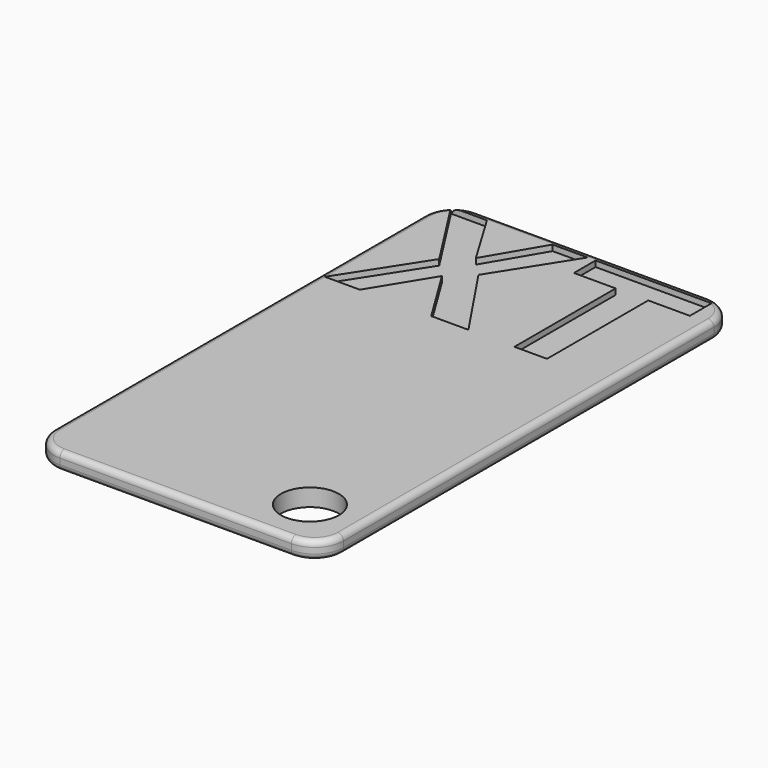
from build123d import *

# Parameters (mm, degrees)
F0_W         = 90
F0_H         = 50
F1_DEPTH     = 3
F2_R         = 1
F3_T1_DEPTH  = 3
F3_T4_ANGLE  = 90
F3_T6_ANGLE  = 90
F3_T8_ANGLE  = 90
F3_T10_ANGLE = 90
F3_T12_ANGLE = 90
F3_T14_ANGLE = 90
F3_T16_ANGLE = 90
F3_T18_ANGLE = 90
F5_ANGLE     = 90
F6_TEXT_SIZE = 37.1822803195
F7_DEPTH     = 1
F8_R         = 5
F9_DEPTH     = 3


# Not quite as in the source:
# - a fillet or chamfer that OpenCascade refuses, or shapes differently, is made with other operations: its cross-section is extruded or revolved along the edge and cut away or added
# - Text() gives the source's letters only with a copy of the font that has no kerning and outlines rounded to 1/6400 em; it was checked with that copy


with BuildPart() as f1:
    # F0 (on Top) → F1 (new body)
    with BuildSketch(Plane.XY):
        Rectangle(F0_W, F0_H)
    extrude(amount=F1_DEPTH)

    # F2
    f2_edges = [f1.edges().sort_by_distance(p)[0] for p in [
        (0, 25, 3),
        (-45, 0, 3),
        (0, -25, 3),
        (45, 0, 3),
        (0, 25, 0),
        (-45, 0, 0),
        (0, -25, 0),
        (45, 0, 0),
    ]]
    fillet(f2_edges, radius=F2_R)

    # F3: fillet of radius 5 on 4 edges, made by hand

    # F3_s2 → F3_t1 (cut)
    with BuildSketch(Plane.XY):
        with BuildLine():
            ThreePointArc((45, -20), (43.5355339059, -23.5355339059), (40, -25))
            Line((40, -25), (45, -25))
            Line((45, -25), (45, -20))
        make_face()
        with BuildLine():
            ThreePointArc((40, 25), (43.5355339059, 23.5355339059), (45, 20))
            Line((45, 20), (45, 25))
            Line((45, 25), (40, 25))
        make_face()
        with BuildLine():
            ThreePointArc((-40, 25), (-43.5355339059, 23.5355339059), (-45, 20))
            Line((-45, 20), (-45, 25))
            Line((-45, 25), (-40, 25))
        make_face()
        with BuildLine():
            ThreePointArc((-45, -20), (-43.5355339059, -23.5355339059), (-40, -25))
            Line((-40, -25), (-45, -25))
            Line((-45, -25), (-45, -20))
        make_face()
    extrude(amount=F3_T1_DEPTH, mode=Mode.SUBTRACT)

    # F3_s3 → F3_t4 (revolve, cut)
    with BuildSketch(Plane.YZ.offset(-40)):
        with BuildLine():
            ThreePointArc((-24, 0), (-24.7071067812, 0.2928932188), (-25, 1))
            Line((-25, 1), (-25, 0))
            Line((-25, 0), (-24, 0))
        make_face()
    revolve(axis=Axis((-40, -20, 0), (0, 0, -1)), revolution_arc=F3_T4_ANGLE, mode=Mode.SUBTRACT)

    # F3_s5 → F3_t6 (revolve, cut)
    with BuildSketch(Plane.XZ.offset(20)):
        with BuildLine():
            ThreePointArc((-44, 3), (-44.7071067812, 2.7071067812), (-45, 2))
            Line((-45, 2), (-45, 3))
            Line((-45, 3), (-44, 3))
        make_face()
    revolve(axis=Axis((-40, -20, 3), (0, 0, 1)), revolution_arc=F3_T6_ANGLE, mode=Mode.SUBTRACT)

    # F3_s7 → F3_t8 (revolve, cut)
    with BuildSketch(Plane.XZ.offset(-20)):
        with BuildLine():
            ThreePointArc((-44, 0), (-44.7071067812, 0.2928932188), (-45, 1))
            Line((-45, 1), (-45, 0))
            Line((-45, 0), (-44, 0))
        make_face()
    revolve(axis=Axis((-40, 20, 0), (0, 0, -1)), revolution_arc=F3_T8_ANGLE, mode=Mode.SUBTRACT)

    # F3_s9 → F3_t10 (revolve, cut)
    with BuildSketch(Plane.YZ.offset(-40)):
        with BuildLine():
            ThreePointArc((24, 3), (24.7071067812, 2.7071067812), (25, 2))
            Line((25, 2), (25, 3))
            Line((25, 3), (24, 3))
        make_face()
    revolve(axis=Axis((-40, 20, 3), (0, 0, 1)), revolution_arc=F3_T10_ANGLE, mode=Mode.SUBTRACT)

    # F3_s11 → F3_t12 (revolve, cut)
    with BuildSketch(Plane.YZ.offset(40)):
        with BuildLine():
            ThreePointArc((24, 0), (24.7071067812, 0.2928932188), (25, 1))
            Line((25, 1), (25, 0))
            Line((25, 0), (24, 0))
        make_face()
    revolve(axis=Axis((40, 20, 0), (0, 0, -1)), revolution_arc=F3_T12_ANGLE, mode=Mode.SUBTRACT)

    # F3_s13 → F3_t14 (revolve, cut)
    with BuildSketch(Plane.XZ.offset(-20)):
        with BuildLine():
            ThreePointArc((44, 3), (44.7071067812, 2.7071067812), (45, 2))
            Line((45, 2), (45, 3))
            Line((45, 3), (44, 3))
        make_face()
    revolve(axis=Axis((40, 20, 3), (0, 0, 1)), revolution_arc=F3_T14_ANGLE, mode=Mode.SUBTRACT)

    # F3_s15 → F3_t16 (revolve, cut)
    with BuildSketch(Plane.XZ.offset(20)):
        with BuildLine():
            ThreePointArc((44, 0), (44.7071067812, 0.2928932188), (45, 1))
            Line((45, 1), (45, 0))
            Line((45, 0), (44, 0))
        make_face()
    revolve(axis=Axis((40, -20, 0), (0, 0, -1)), revolution_arc=F3_T16_ANGLE, mode=Mode.SUBTRACT)

    # F3_s17 → F3_t18 (revolve, cut)
    with BuildSketch(Plane.YZ.offset(40)):
        with BuildLine():
            ThreePointArc((-24, 3), (-24.7071067812, 2.7071067812), (-25, 2))
            Line((-25, 2), (-25, 3))
            Line((-25, 3), (-24, 3))
        make_face()
    revolve(axis=Axis((40, -20, 3), (0, 0, 1)), revolution_arc=F3_T18_ANGLE, mode=Mode.SUBTRACT)


with BuildPart() as f1_1:
    # F5: moved
    add(f1.part.rotate(Axis((0, 0, 16.4477843791), (0, 0, 1)), F5_ANGLE))

    # F6 (on face) → F7 (cut)
    with BuildSketch(Plane.XY.offset(3)):
        with Locations((-24, 17.2287581699)):
            Text('XT', F6_TEXT_SIZE, font='Open Sans', font_style=FontStyle.BOLD, text_align=(TextAlign.LEFT, TextAlign.BOTTOM))
    extrude(amount=-F7_DEPTH, mode=Mode.SUBTRACT)

    # F8 (on face) → F9 (cut)
    with BuildSketch(Plane.XY.offset(3)):
        with Locations((16, -36)):
            Circle(F8_R)
    extrude(amount=-F9_DEPTH, mode=Mode.SUBTRACT)


solid = f1_1.part
